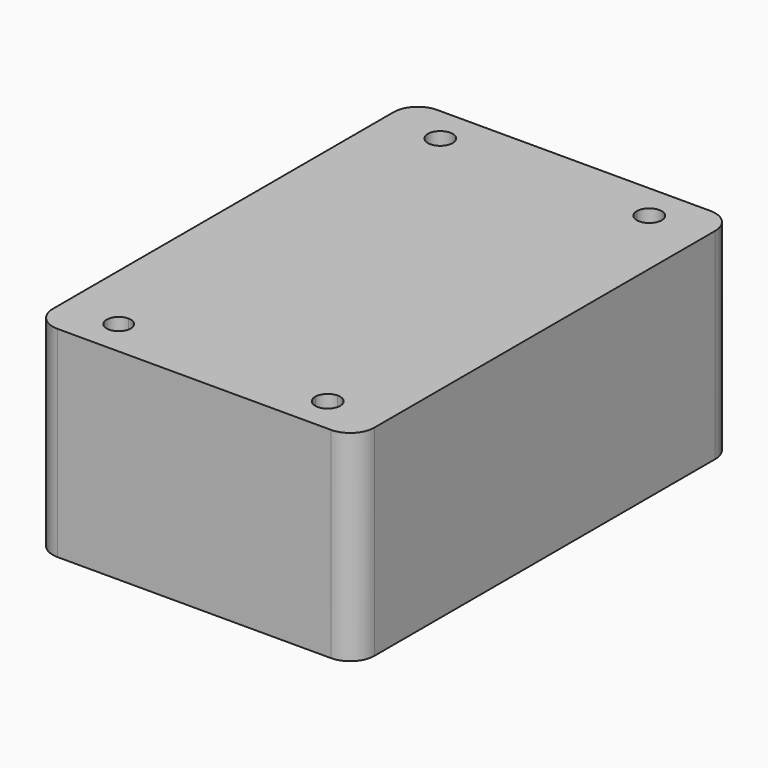
from build123d import *

# Parameters (mm, degrees)
F0_W     = 40
F0_H     = 59
F1_DEPTH = 25
F2_R     = 3


with BuildPart() as f1:
    # F0 (on Top) → F1 (new body)
    with BuildSketch(Plane.XY):
        Rectangle(F0_W, F0_H)
        with BuildLine():
            ThreePointArc((-13, 23.45), (-14.0960155108, 26.0960155108), (-11.45, 25))
            Line((-11.45, 25), (11.45, 25))
            ThreePointArc((11.45, 25), (13, 26.55), (14.55, 25))
            ThreePointArc((14.55, 25), (14.0960155108, 23.9039844892), (13, 23.45))
            Line((13, 23.45), (13, -23.45))
            ThreePointArc((13, -23.45), (14.0960155108, -23.9039844892), (14.55, -25))
            ThreePointArc((14.55, -25), (13, -26.55), (11.45, -25))
            Line((11.45, -25), (-11.5, -25))
            ThreePointArc((-11.5, -25), (-14.0606601718, -26.0606601718), (-13, -23.5))
            Line((-13, -23.5), (-13, 23.45))
        make_face(mode=Mode.SUBTRACT)
        with BuildLine():
            Line((11.45, 25), (-11.45, 25))
            ThreePointArc((-11.45, 25), (-11.9039844892, 23.9039844892), (-13, 23.45))
            Line((-13, 23.45), (-13, -23.5))
            ThreePointArc((-13, -23.5), (-11.9393398282, -23.9393398282), (-11.5, -25))
            Line((-11.5, -25), (11.45, -25))
            ThreePointArc((11.45, -25), (11.9039844892, -23.9039844892), (13, -23.45))
            Line((13, -23.45), (13, 23.45))
            ThreePointArc((13, 23.45), (11.9039844892, 23.9039844892), (11.45, 25))
        make_face()
    extrude(amount=F1_DEPTH)

    # F2
    f2_edges = [f1.edges().sort_by_distance(p)[0] for p in [
        (-20, 29.5, 12.5),
        (20, 29.5, 12.5),
        (20, -29.5, 12.5),
        (-20, -29.5, 12.5),
    ]]
    fillet(f2_edges, radius=F2_R)


solid = f1.part
